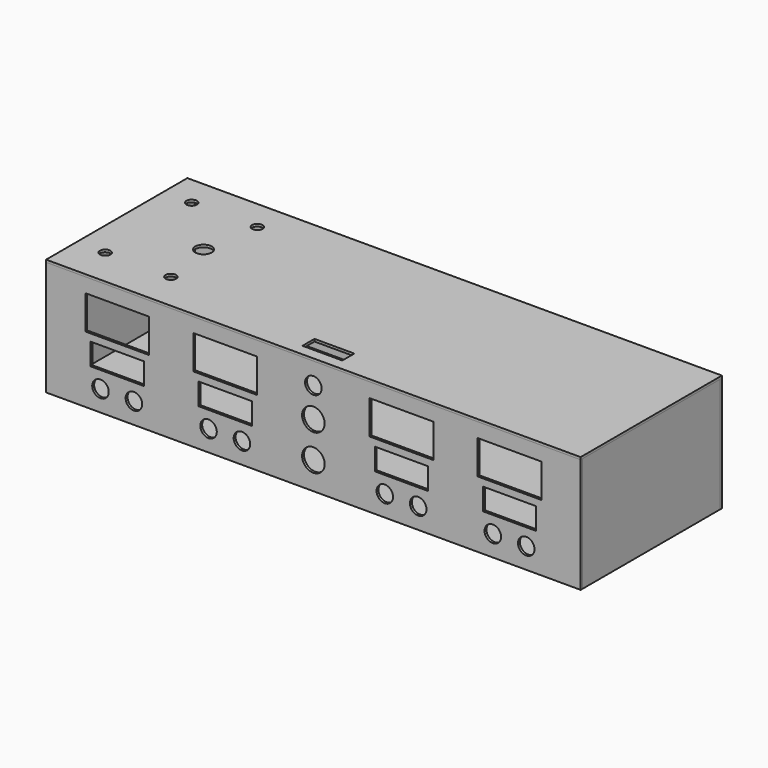
from build123d import *

# Parameters (mm, degrees)
F0_W     = 12.7
F0_H     = 12.7
F0_W_2   = 685.8
F0_H_2   = 139.7
F0_R     = 11
F0_W_3   = 71
F0_H_3   = 29
F0_R_2   = 15
F0_W_4   = 85
F0_H_4   = 45
F1_DEPTH = 3.175
F2_DEPTH = 228.6
F3_W     = 685.8
F3_H     = 139.7
F3_R     = 11.1125
F4_DEPTH = 3.175
F5_W     = 12.7
F5_H     = 228.6
F5_R     = 7
F5_W_2   = 53
F5_H_2   = 20
F5_R_2   = 11
F6_DEPTH = 3.175


# Not quite as in the source:
# - a feature names something its author has since deleted; it is built from what else it names


with BuildPart() as f1:
    # F0 (on Front) → F1 (new body)
    with BuildSketch(Plane.XZ):
        with Locations((6.35, 6.35)):
            Rectangle(F0_W, F0_H)
        with Locations((355.6, 6.35)):
            Rectangle(F0_W_2, F0_H)
        with Locations((704.85, 6.35)):
            Rectangle(F0_W, F0_H)
        with Locations((6.35, 82.55)):
            Rectangle(F0_W, F0_H_2)
        with Locations((355.6, 82.55)):
            Rectangle(F0_W_2, F0_H_2)
        with Locations((72.39, 27.7125)):
            Circle(F0_R, mode=Mode.SUBTRACT)
        with Locations((116.84, 27.7125)):
            Circle(F0_R, mode=Mode.SUBTRACT)
        with Locations((216.1286, 27.7125)):
            Circle(F0_R, mode=Mode.SUBTRACT)
        with Locations((260.5786, 27.7125)):
            Circle(F0_R, mode=Mode.SUBTRACT)
        with Locations((94.615, 64.325)):
            Rectangle(F0_W_3, F0_H_3, mode=Mode.SUBTRACT)
        with Locations((238.3536, 64.325)):
            Rectangle(F0_W_3, F0_H_3, mode=Mode.SUBTRACT)
        with Locations((355.6, 36.5125)):
            Circle(F0_R_2, mode=Mode.SUBTRACT)
        with Locations((450.6214, 27.7125)):
            Circle(F0_R, mode=Mode.SUBTRACT)
        with Locations((495.0714, 27.7125)):
            Circle(F0_R, mode=Mode.SUBTRACT)
        with Locations((594.36, 27.7125)):
            Circle(F0_R, mode=Mode.SUBTRACT)
        with Locations((638.81, 27.7125)):
            Circle(F0_R, mode=Mode.SUBTRACT)
        with Locations((472.8464, 64.325)):
            Rectangle(F0_W_3, F0_H_3, mode=Mode.SUBTRACT)
        with Locations((616.585, 64.325)):
            Rectangle(F0_W_3, F0_H_3, mode=Mode.SUBTRACT)
        with Locations((94.615, 110.85)):
            Rectangle(F0_W_4, F0_H_4, mode=Mode.SUBTRACT)
        with Locations((238.3536, 110.85)):
            Rectangle(F0_W_4, F0_H_4, mode=Mode.SUBTRACT)
        with Locations((355.6, 84.1375)):
            Circle(F0_R_2, mode=Mode.SUBTRACT)
        with Locations((472.8464, 110.85)):
            Rectangle(F0_W_4, F0_H_4, mode=Mode.SUBTRACT)
        with Locations((616.585, 110.85)):
            Rectangle(F0_W_4, F0_H_4, mode=Mode.SUBTRACT)
        with Locations((355.6, 123.825)):
            Circle(F0_R, mode=Mode.SUBTRACT)
        with Locations((704.85, 82.55)):
            Rectangle(F0_W, F0_H_2)
    extrude(amount=F1_DEPTH)


with BuildPart() as f2:
    # F0 (on Front) → F2 (new body)
    with BuildSketch(Plane.XZ):
        with Locations((355.6, 6.35)):
            Rectangle(F0_W_2, F0_H)
        with Locations((6.35, 6.35)):
            Rectangle(F0_W, F0_H)
        with Locations((704.85, 6.35)):
            Rectangle(F0_W, F0_H)
        with Locations((6.35, 82.55)):
            Rectangle(F0_W, F0_H_2)
        with Locations((704.85, 82.55)):
            Rectangle(F0_W, F0_H_2)
    extrude(amount=-F2_DEPTH)


with BuildPart() as f4:
    # F3 (on face) → F4 (new body)
    with BuildSketch(Plane(origin=(0, 228.6, 0), x_dir=(-1, 0, 0), z_dir=(0, 1, 0))):
        Polygon((-711.2, 152.4), (-711.2, 0), (0, 0), (0, 152.4), (-12.7, 152.4), (-12.7, 12.7), (-698.5, 12.7), (-698.5, 152.4), align=None)
        with Locations((-355.6, 82.55)):
            Rectangle(F3_W, F3_H)
        with Locations((-634.085, 76.2)):
            Circle(F3_R, mode=Mode.SUBTRACT)
        with Locations((-599.085, 76.2)):
            Circle(F3_R, mode=Mode.SUBTRACT)
        with Locations((-490.3464, 76.2)):
            Circle(F3_R, mode=Mode.SUBTRACT)
        with Locations((-455.3464, 76.2)):
            Circle(F3_R, mode=Mode.SUBTRACT)
        with Locations((-355.6, 76.2)):
            Circle(F3_R, mode=Mode.SUBTRACT)
        with Locations((-255.8536, 76.2)):
            Circle(F3_R, mode=Mode.SUBTRACT)
        with Locations((-220.8536, 76.2)):
            Circle(F3_R, mode=Mode.SUBTRACT)
        with Locations((-112.115, 76.2)):
            Circle(F3_R, mode=Mode.SUBTRACT)
        with Locations((-77.115, 76.2)):
            Circle(F3_R, mode=Mode.SUBTRACT)
    extrude(amount=F4_DEPTH)


with BuildPart() as f6:
    # F5 (on face) → F6 (new body)
    with BuildSketch(Plane.XY.offset(152.4)):
        with Locations((6.35, 114.3)):
            Rectangle(F5_W, F5_H)
        Polygon((12.7, 0), (0, 0), (0, -3.175), (711.2, -3.175), (711.2, 0), (711.2, 228.6), (711.2, 231.775), (0, 231.775), (0, 228.6), (12.7, 228.6), align=None)
        with Locations((38.1032319846, 47.4996870108)):
            Circle(F5_R, mode=Mode.SUBTRACT)
        with Locations((125.4632319846, 47.4996870108)):
            Circle(F5_R, mode=Mode.SUBTRACT)
        with Locations((355.6, 21.825)):
            Rectangle(F5_W_2, F5_H_2, mode=Mode.SUBTRACT)
        with Locations((113.4632319846, 116.7996870108)):
            Circle(F5_R_2, mode=Mode.SUBTRACT)
        with Locations((38.1032319846, 191.2996870108)):
            Circle(F5_R, mode=Mode.SUBTRACT)
        with Locations((125.4632319846, 191.2996870108)):
            Circle(F5_R, mode=Mode.SUBTRACT)
    extrude(amount=F6_DEPTH)


solid = Compound([f1.part, f2.part, f4.part, f6.part])
